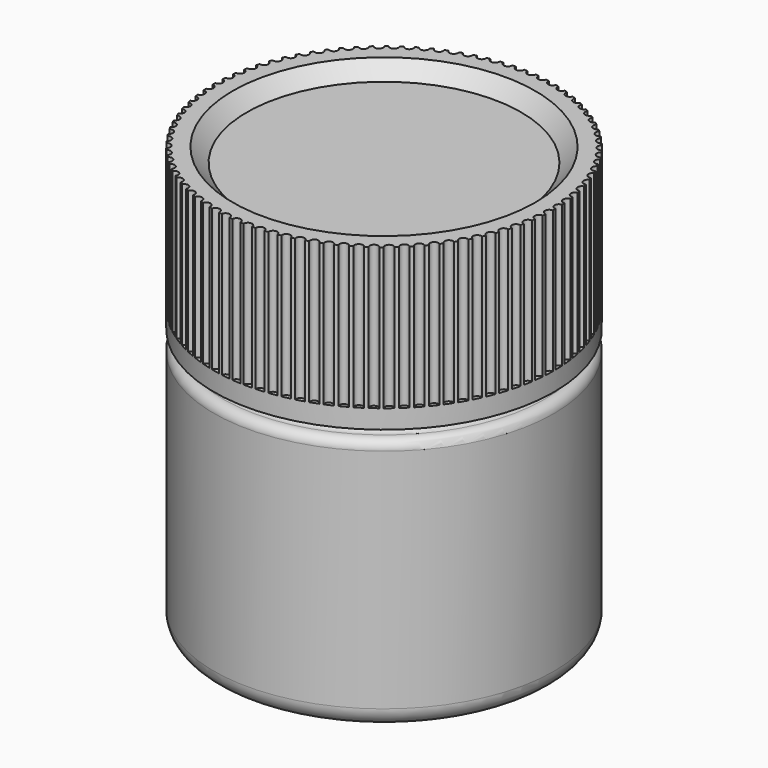
from build123d import *

# Parameters (mm, degrees)
F0_R      = 18
F1_DEPTH  = 27
F2_R      = 16
F3_DEPTH  = 1
F4_R      = 18
F5_DEPTH  = 17
F6_R      = 2
F7_R      = 0.99999
F8_R      = 16
F9_DEPTH  = 1.5
F9_TAPER  = 45
F10_R     = 0.45
F11_DEPTH = 15


# Not quite as in the source:
# - a fillet or chamfer is up to 0.001 mm smaller than in the source, because OpenCascade refuses the exact size


with BuildPart() as f1:
    # F0 (on Top) → F1 (new body)
    with BuildSketch(Plane.XY):
        Circle(F0_R)
    extrude(amount=F1_DEPTH)

    # F2 (on face) → F3 (join)
    with BuildSketch(Plane.XY.offset(27)):
        Circle(F2_R)
    extrude(amount=F3_DEPTH)

    # F4 (on face) → F5 (join)
    with BuildSketch(Plane.XY.offset(28)):
        Circle(F4_R)
    extrude(amount=F5_DEPTH)

    # F6
    f6_edges = [f1.edges().sort_by_distance(p)[0] for p in [
        (-18, 0, 0),
    ]]
    fillet(f6_edges, radius=F6_R)

    # F7 (radius 1 in the source; OpenCascade refuses exactly that, so slightly less here)
    f7_edges = [f1.edges().sort_by_distance(p)[0] for p in [
        (-18, 0, 27),
        (-16, 0, 27),
    ]]
    fillet(f7_edges, radius=F7_R)

    # F8 (on face) → F9 (cut)
    with BuildSketch(Plane.XY.offset(45)):
        Circle(F8_R)
    extrude(amount=-F9_DEPTH, taper=F9_TAPER, mode=Mode.SUBTRACT)

    # F10 (on face) → F11 (cut)
    with BuildSketch(Plane.XY.offset(45)):
        with Locations((0, 18)):
            Circle(F10_R)
        with Locations((-1.2556165274, 17.9561529047)):
            Circle(F10_R)
        with Locations((-2.5051158173, 17.8248252373)):
            Circle(F10_R)
        with Locations((-3.7424104347, 17.6066568132)):
            Circle(F10_R)
        with Locations((-4.9614724047, 17.3027105269)):
            Circle(F10_R)
        with Locations((-6.1563625799, 16.9144671741)):
            Circle(F10_R)
        with Locations((-7.3212595754, 16.4438182376)):
            Circle(F10_R)
        with Locations((-8.4504881301, 15.8930566715)):
            Circle(F10_R)
        with Locations((-9.5385467562, 15.2648657308)):
            Circle(F10_R)
        with Locations((-10.5801345413, 14.5623058987)):
            Circle(F10_R)
        with Locations((-11.5701769744, 13.7887999761)):
            Circle(F10_R)
        with Locations((-12.5038506683, 12.9481164061)):
            Circle(F10_R)
        with Locations((-13.3766068586, 12.0443509145)):
            Circle(F10_R)
        with Locations((-14.1841935649, 11.0819065559)):
            Circle(F10_R)
        with Locations((-14.922676306, 10.0654722625)):
            Circle(F10_R)
        with Locations((-15.5884572681, 9)):
            Circle(F10_R)
        with Locations((-16.1782928334, 7.8906806422)):
            Circle(F10_R)
        with Locations((-16.6893093822, 6.7429186815)):
            Circle(F10_R)
        with Locations((-17.1190172933, 5.5623058987)):
            Circle(F10_R)
        with Locations((-17.465323073, 4.3545941208)):
            Circle(F10_R)
        with Locations((-17.7265395542, 3.125667198)):
            Circle(F10_R)
        with Locations((-17.9013941166, 1.8815123388)):
            Circle(F10_R)
        with Locations((-17.9890348863, 0.6281909406)):
            Circle(F10_R)
        with Locations((-17.9890348863, -0.6281909406)):
            Circle(F10_R)
        with Locations((-17.9013941166, -1.8815123388)):
            Circle(F10_R)
        with Locations((-17.7265395542, -3.125667198)):
            Circle(F10_R)
        with Locations((-17.465323073, -4.3545941208)):
            Circle(F10_R)
        with Locations((-17.1190172933, -5.5623058987)):
            Circle(F10_R)
        with Locations((-16.6893093822, -6.7429186815)):
            Circle(F10_R)
        with Locations((-16.1782928334, -7.8906806422)):
            Circle(F10_R)
        with Locations((-15.5884572681, -9)):
            Circle(F10_R)
        with Locations((-14.922676306, -10.0654722625)):
            Circle(F10_R)
        with Locations((-14.1841935649, -11.0819065559)):
            Circle(F10_R)
        with Locations((-13.3766068586, -12.0443509145)):
            Circle(F10_R)
        with Locations((-12.5038506683, -12.9481164061)):
            Circle(F10_R)
        with Locations((-11.5701769744, -13.7887999761)):
            Circle(F10_R)
        with Locations((-10.5801345413, -14.5623058987)):
            Circle(F10_R)
        with Locations((-9.5385467562, -15.2648657308)):
            Circle(F10_R)
        with Locations((-8.4504881301, -15.8930566715)):
            Circle(F10_R)
        with Locations((-7.3212595754, -16.4438182376)):
            Circle(F10_R)
        with Locations((-6.1563625799, -16.9144671741)):
            Circle(F10_R)
        with Locations((-4.9614724047, -17.3027105269)):
            Circle(F10_R)
        with Locations((-3.7424104347, -17.6066568132)):
            Circle(F10_R)
        with Locations((-2.5051158173, -17.8248252373)):
            Circle(F10_R)
        with Locations((-1.2556165274, -17.9561529047)):
            Circle(F10_R)
        with Locations((0, -18)):
            Circle(F10_R)
        with Locations((1.2556165274, -17.9561529047)):
            Circle(F10_R)
        with Locations((2.5051158173, -17.8248252373)):
            Circle(F10_R)
        with Locations((3.7424104347, -17.6066568132)):
            Circle(F10_R)
        with Locations((4.9614724047, -17.3027105269)):
            Circle(F10_R)
        with Locations((6.1563625799, -16.9144671741)):
            Circle(F10_R)
        with Locations((7.3212595754, -16.4438182376)):
            Circle(F10_R)
        with Locations((8.4504881301, -15.8930566715)):
            Circle(F10_R)
        with Locations((9.5385467562, -15.2648657308)):
            Circle(F10_R)
        with Locations((10.5801345413, -14.5623058987)):
            Circle(F10_R)
        with Locations((11.5701769744, -13.7887999761)):
            Circle(F10_R)
        with Locations((12.5038506683, -12.9481164061)):
            Circle(F10_R)
        with Locations((13.3766068586, -12.0443509145)):
            Circle(F10_R)
        with Locations((14.1841935649, -11.0819065559)):
            Circle(F10_R)
        with Locations((14.922676306, -10.0654722625)):
            Circle(F10_R)
        with Locations((15.5884572681, -9)):
            Circle(F10_R)
        with Locations((16.1782928334, -7.8906806422)):
            Circle(F10_R)
        with Locations((16.6893093822, -6.7429186815)):
            Circle(F10_R)
        with Locations((17.1190172933, -5.5623058987)):
            Circle(F10_R)
        with Locations((17.465323073, -4.3545941208)):
            Circle(F10_R)
        with Locations((17.7265395542, -3.125667198)):
            Circle(F10_R)
        with Locations((17.9013941166, -1.8815123388)):
            Circle(F10_R)
        with Locations((17.9890348863, -0.6281909406)):
            Circle(F10_R)
        with Locations((17.9890348863, 0.6281909406)):
            Circle(F10_R)
        with Locations((17.9013941166, 1.8815123388)):
            Circle(F10_R)
        with Locations((17.7265395542, 3.125667198)):
            Circle(F10_R)
        with Locations((17.465323073, 4.3545941208)):
            Circle(F10_R)
        with Locations((17.1190172933, 5.5623058987)):
            Circle(F10_R)
        with Locations((16.6893093822, 6.7429186815)):
            Circle(F10_R)
        with Locations((16.1782928334, 7.8906806422)):
            Circle(F10_R)
        with Locations((15.5884572681, 9)):
            Circle(F10_R)
        with Locations((14.922676306, 10.0654722625)):
            Circle(F10_R)
        with Locations((14.1841935649, 11.0819065559)):
            Circle(F10_R)
        with Locations((13.3766068586, 12.0443509145)):
            Circle(F10_R)
        with Locations((12.5038506683, 12.9481164061)):
            Circle(F10_R)
        with Locations((11.5701769744, 13.7887999761)):
            Circle(F10_R)
        with Locations((10.5801345413, 14.5623058987)):
            Circle(F10_R)
        with Locations((9.5385467562, 15.2648657308)):
            Circle(F10_R)
        with Locations((8.4504881301, 15.8930566715)):
            Circle(F10_R)
        with Locations((7.3212595754, 16.4438182376)):
            Circle(F10_R)
        with Locations((6.1563625799, 16.9144671741)):
            Circle(F10_R)
        with Locations((4.9614724047, 17.3027105269)):
            Circle(F10_R)
        with Locations((3.7424104347, 17.6066568132)):
            Circle(F10_R)
        with Locations((2.5051158173, 17.8248252373)):
            Circle(F10_R)
        with Locations((1.2556165274, 17.9561529047)):
            Circle(F10_R)
    extrude(amount=-F11_DEPTH, mode=Mode.SUBTRACT)


solid = f1.part
